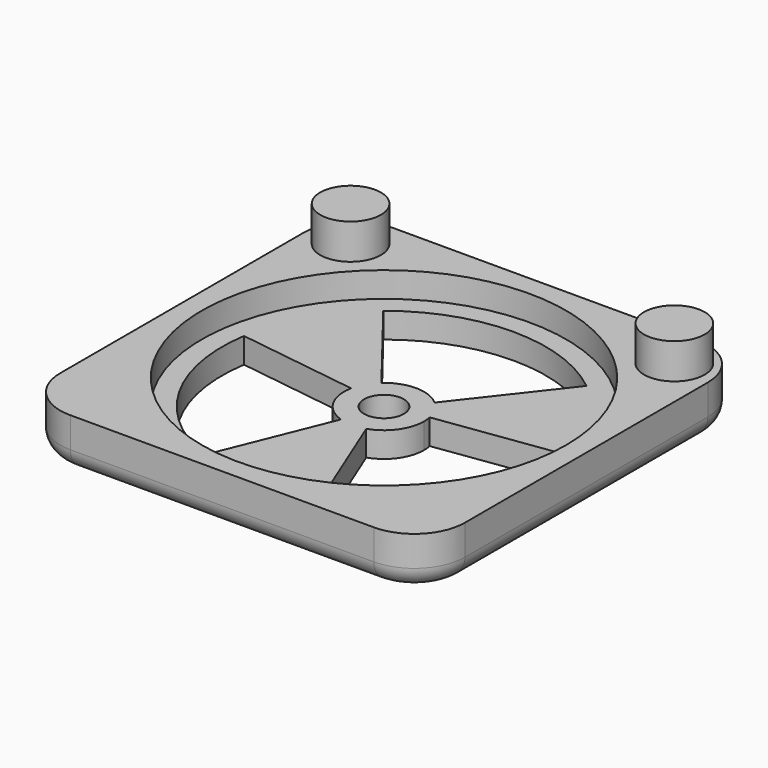
from build123d import *

# Parameters (mm, degrees)
F0_W     = 40
F0_H     = 40
F0_R     = 3
F0_R_2   = 18
F1_DEPTH = 5
F2_DEPTH = 8.5
F3_R     = 5
F4_R     = 1.99999
F0_R_3   = 1.96412235
F5_DEPTH = 2.5


# Not quite as in the source:
# - a fillet or chamfer is up to 0.001 mm smaller than in the source, because OpenCascade refuses the exact size


with BuildPart() as f1:
    # F0 (on Top) → F1 (new body)
    with BuildSketch(Plane.XY):
        Rectangle(F0_W, F0_H)
        with Locations((-16, 15.8712012513)):
            Circle(F0_R, mode=Mode.SUBTRACT)
        Circle(F0_R_2, mode=Mode.SUBTRACT)
        with Locations((16, 15.8712012513)):
            Circle(F0_R, mode=Mode.SUBTRACT)
    extrude(amount=F1_DEPTH)

    # F0 (on Top) → F2 (join)
    with BuildSketch(Plane.XY):
        with Locations((-16, 15.8712012513)):
            Circle(F0_R)
        with Locations((16, 15.8712012513)):
            Circle(F0_R)
    extrude(amount=F2_DEPTH)

    # F3
    f3_edges = [f1.edges().sort_by_distance(p)[0] for p in [
        (-20, -20, 2.5),
        (-20, 20, 2.5),
        (20, -20, 2.5),
        (20, 20, 2.5),
    ]]
    fillet(f3_edges, radius=F3_R)

    # F4 (radius 2 in the source; OpenCascade refuses exactly that, so slightly less here)
    f4_edges = [f1.edges().sort_by_distance(p)[0] for p in [
        (20, 0, 0),
    ]]
    fillet(f4_edges, radius=F4_R)

    # F0 (on Top) → F5 (join)
    with BuildSketch(Plane.XY):
        Circle(F0_R_2)
        with BuildLine():
            ThreePointArc((15.8087915907, 2.4661931072), (15.952126276, 1.236797184), (16, 0))
            ThreePointArc((16, 0), (13.1965480074, -9.0471609187), (5.7686099139, -14.9239116743))
            ThreePointArc((5.7686099139, -14.9239116743), (0, -16), (-5.7686099139, -14.9239116743))
            ThreePointArc((-5.7686099139, -14.9239116743), (-13.8564064606, -8), (-15.8087915907, 2.4661931072))
            ThreePointArc((-15.8087915907, 2.4661931072), (-13.8564064606, 8), (-10.0401816768, 12.4577185671))
            ThreePointArc((-10.0401816768, 12.4577185671), (0, 16), (10.0401816768, 12.4577185671))
            ThreePointArc((10.0401816768, 12.4577185671), (13.8564064606, 8), (15.8087915907, 2.4661931072))
        make_face(mode=Mode.SUBTRACT)
        with BuildLine():
            ThreePointArc((3.96412235, 0), (3.9439266403, 0.3996356611), (3.8835452903, 0.795199336))
            ThreePointArc((3.8835452903, 0.795199336), (3.4330306588, 1.982061175), (2.6304354712, 2.9656492102))
            ThreePointArc((2.6304354712, 2.9656492102), (0, 3.96412235), (-2.6304354712, 2.9656492102))
            ThreePointArc((-2.6304354712, 2.9656492102), (-3.4330306588, 1.982061175), (-3.8835452903, 0.795199336))
            ThreePointArc((-3.8835452903, 0.795199336), (-3.4330306588, -1.982061175), (-1.2531098191, -3.7608485461))
            ThreePointArc((-1.2531098191, -3.7608485461), (0, -3.96412235), (1.2531098191, -3.7608485461))
            ThreePointArc((1.2531098191, -3.7608485461), (3.2157228306, -2.3180579549), (3.96412235, 0))
        make_face()
        Circle(F0_R_3, mode=Mode.SUBTRACT)
        with BuildLine():
            ThreePointArc((-5.7686099139, -14.9239116743), (0, -16), (5.7686099139, -14.9239116743))
            Line((5.7686099139, -14.9239116743), (1.2531098191, -3.7608485461))
            ThreePointArc((1.2531098191, -3.7608485461), (0, -3.96412235), (-1.2531098191, -3.7608485461))
            Line((-1.2531098191, -3.7608485461), (-5.7686099139, -14.9239116743))
        make_face()
        with BuildLine():
            Line((3.8835452903, 0.795199336), (15.8087915907, 2.4661931072))
            ThreePointArc((15.8087915907, 2.4661931072), (13.8564064606, 8), (10.0401816768, 12.4577185671))
            Line((10.0401816768, 12.4577185671), (2.6304354712, 2.9656492102))
            ThreePointArc((2.6304354712, 2.9656492102), (3.4330306588, 1.982061175), (3.8835452903, 0.795199336))
        make_face()
        with BuildLine():
            Line((-2.6304354712, 2.9656492102), (-10.0401816768, 12.4577185671))
            ThreePointArc((-10.0401816768, 12.4577185671), (-13.8564064606, 8), (-15.8087915907, 2.4661931072))
            Line((-15.8087915907, 2.4661931072), (-3.8835452903, 0.795199336))
            ThreePointArc((-3.8835452903, 0.795199336), (-3.4330306588, 1.982061175), (-2.6304354712, 2.9656492102))
        make_face()
    extrude(amount=F5_DEPTH)


solid = f1.part
